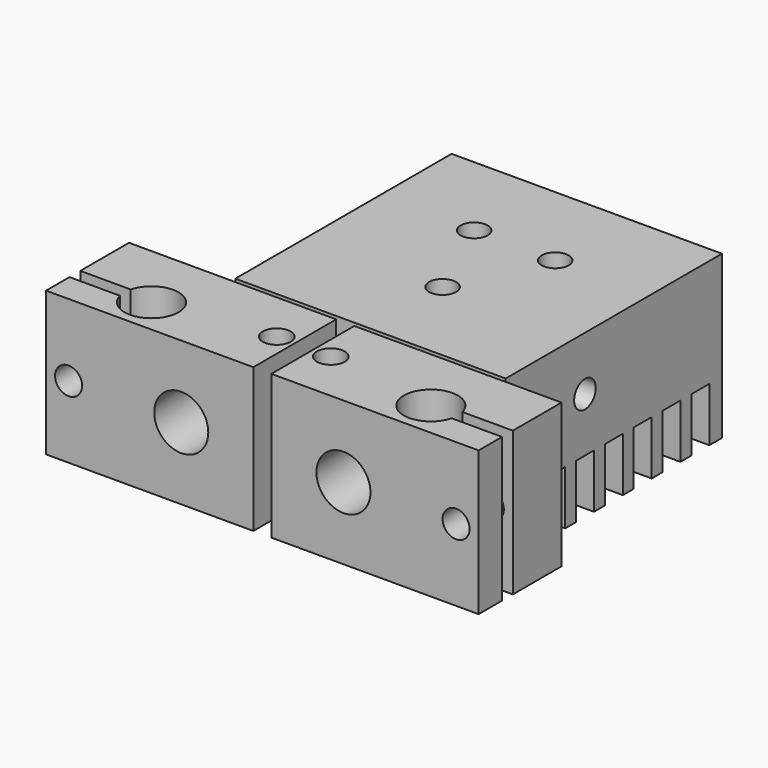
from build123d import *

# Parameters (mm, degrees)
F0_W      = 30
F0_H      = 30
F15_DEPTH = 18
F1_D      = 8
F1_DEPTH  = 6.5
F1_TIP    = 2.4034424761
F17_W     = 30
F17_H     = 2.5
F18_DEPTH = 6
F19_D     = 3
F19_DEPTH = 10
F19_TIP   = 0.9012909285
F2_R      = 1.475
F3_DEPTH  = 3.5
F20_W     = 23
F20_H     = 16
F21_DEPTH = 11.5
F22_R     = 3
F5_DEPTH  = 6
F22_R_2   = 1.5
F6_DEPTH  = 11.5
F7_R      = 1.55
F23_DEPTH = 16
F8_R      = 1.5
F9_DEPTH  = 8
F10_DEPTH = 6
F11_R     = 1.5
F12_DEPTH = 6


# Not quite as in the source:
# - a feature names something its author has since deleted; it is built from what else it names


with BuildPart() as f15:
    # F0 (on Top) → F15 (new body)
    with BuildSketch(Plane.XY):
        Rectangle(F0_W, F0_H)
    extrude(amount=F15_DEPTH)

    # F1
    with Locations(Plane(origin=(0, 15, 0), x_dir=(-1, 0, 0), z_dir=(0, 1, 0))):
        with Locations((-9, 12), (9, 12)):
            Hole(F1_D / 2, depth=F1_DEPTH)
            with Locations((0, 0, -(F1_DEPTH + F1_TIP / 2))):  # 118° drill point
                Cone(0, F1_D / 2, F1_TIP, mode=Mode.SUBTRACT)

    # F17 (on face) → F18 (cut)
    with BuildSketch(Plane(origin=(0, 0, 0), x_dir=(1, 0, 0), z_dir=(0, 0, -1))):
        with Locations((0, 12)):
            Rectangle(F17_W, F17_H)
        with Locations((0, 8)):
            Rectangle(F17_W, F17_H)
        with Locations((0, 4)):
            Rectangle(F17_W, F17_H)
        Rectangle(F17_W, F17_H)
        with Locations((0, -4)):
            Rectangle(F17_W, F17_H)
        with Locations((0, -8)):
            Rectangle(F17_W, F17_H)
        with Locations((0, -12)):
            Rectangle(F17_W, F17_H)
    extrude(amount=-F18_DEPTH, mode=Mode.SUBTRACT)

    # F19
    with Locations(Plane(origin=(0, 15, 0), x_dir=(-1, 0, 0), z_dir=(0, 1, 0))):
        with Locations((8.5, 3), (-8.5, 3), (0, 15)):
            Hole(F19_D / 2, depth=F19_DEPTH)
            with Locations((0, 0, -(F19_DEPTH + F19_TIP / 2))):  # 118° drill point
                Cone(0, F19_D / 2, F19_TIP, mode=Mode.SUBTRACT)

    # F2 (on face) → F3 (join)
    with BuildSketch(Plane.XZ.offset(15)):
        with Locations((-9, 12)):
            Circle(F2_R)
        with Locations((9, 12)):
            Circle(F2_R)
    extrude(amount=F3_DEPTH)

    # F20 (on offset) → F21 (join)
    with BuildSketch(Plane.XZ.offset(18.5)):
        with Locations((-12.5, 12)):
            Rectangle(F20_W, F20_H)
        with Locations((12.5, 12)):
            Rectangle(F20_W, F20_H)
    extrude(amount=F21_DEPTH)

    # F22 (on face) → F5 (cut)
    with BuildSketch(Plane.XZ.offset(30)):
        with Locations((-9, 12)):
            Circle(F22_R)
        with Locations((9, 12)):
            Circle(F22_R)
    extrude(amount=-F5_DEPTH, mode=Mode.SUBTRACT)

    # F22 (on face) → F6 (cut, through all)
    with BuildSketch(Plane.XZ.offset(30)):
        with Locations((-21.5, 12)):
            Circle(F22_R_2)
        with Locations((21.5, 12)):
            Circle(F22_R_2)
    extrude(amount=-F6_DEPTH, mode=Mode.SUBTRACT)

    # F7 (on face) → F23 (cut, through all)
    with BuildSketch(Plane.XY.offset(20)):
        with BuildLine():
            Line((-24, -26.75), (-18.4047375097, -26.75))
            ThreePointArc((-18.4047375097, -26.75), (-12.5, -26), (-18.4047375097, -25.25))
            Line((-18.4047375097, -25.25), (-24, -25.25))
            Line((-24, -25.25), (-24, -26.75))
        make_face()
        with Locations((-3, -24.25)):
            Circle(F7_R)
        with Locations((3, -24.25)):
            Circle(F7_R)
        with BuildLine():
            Line((18.4047375097, -26.75), (24, -26.75))
            Line((24, -26.75), (24, -25.25))
            Line((24, -25.25), (18.4047375097, -25.25))
            ThreePointArc((18.4047375097, -25.25), (12.5, -26), (18.4047375097, -26.75))
        make_face()
    extrude(amount=-F23_DEPTH, mode=Mode.SUBTRACT)

    # F8 (on face) → F9 (cut)
    with BuildSketch(Plane.XY.offset(18)):
        with Locations((0, -5)):
            Circle(F8_R)
        with Locations((4.5, 5)):
            Circle(F8_R)
        with Locations((-4.5, 5)):
            Circle(F8_R)
    extrude(amount=-F9_DEPTH, mode=Mode.SUBTRACT)

    # F22 (on face) → F10 (cut)
    with BuildSketch(Plane.XZ.offset(30)):
        with Locations((-9, 12)):
            Circle(F22_R)
    extrude(amount=-F10_DEPTH, mode=Mode.SUBTRACT)

    # F13: F12b, F12 across plane


with BuildPart() as f12:
    # F11 (on face) → F12 (new body)
    with BuildSketch(Plane.YZ.offset(15)):
        with Locations((-12, 12)):
            Circle(F11_R)
    extrude(amount=-F12_DEPTH)


with BuildPart() as f12b:
    # F11 (on face) → F12, piece 2 (new body)
    with BuildSketch(Plane.YZ.offset(15)):
        with Locations((-4, 12)):
            Circle(F11_R)
    extrude(amount=-F12_DEPTH)


with BuildPart() as f15_1:
    add(f15.part)
    add(f12b.part.mirror(Plane.YZ), mode=Mode.SUBTRACT)
    add(f12.part.mirror(Plane.YZ), mode=Mode.SUBTRACT)

    # F14: cut F12, F12b
    add(f12.part, mode=Mode.SUBTRACT)
    add(f12b.part, mode=Mode.SUBTRACT)


solid = f15_1.part
